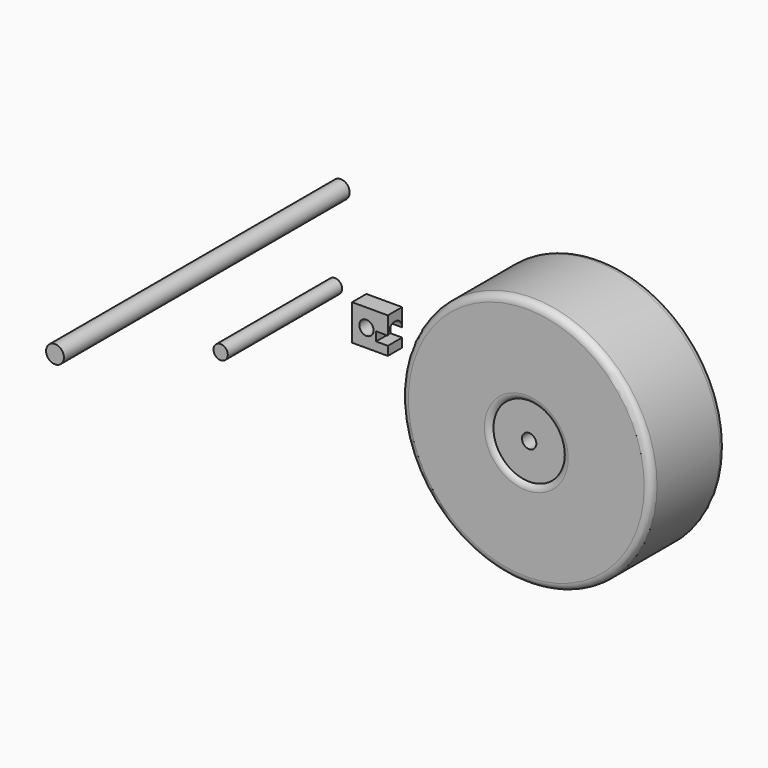
from build123d import *

# Parameters (mm, degrees)
F0_R     = 10
F0_R_2   = 2
F1_DEPTH = 12
F0_R_3   = 35
F2_DEPTH = 13
F4_R     = 2.5
F5_DEPTH = 100
F4_R_2   = 2
F6_DEPTH = 40
F4_W     = 3.3058956834
F4_H     = 1
F4_H_2   = 2.5
F7_DEPTH = 2.5


# Not quite as in the source:
# - a fillet or chamfer that OpenCascade refuses, or shapes differently, is made with other operations: its cross-section is extruded or revolved along the edge and cut away or added


with BuildPart() as f1:
    # F0 (on Front) → F1 (new body, symmetric)
    with BuildSketch(Plane.XZ):
        Circle(F0_R)
        Circle(F0_R_2, mode=Mode.SUBTRACT)
    extrude(amount=F1_DEPTH, both=True)

    # F0 (on Front) → F2 (join, symmetric)
    with BuildSketch(Plane.XZ):
        Circle(F0_R_3)
        Circle(F0_R, mode=Mode.SUBTRACT)
    extrude(amount=F2_DEPTH, both=True)

    # F3: fillet of radius 2 on 4 edges, made by hand

    # F3_s1 → F3_t2 (revolve, cut)
    with BuildSketch(Plane.XY):
        with BuildLine():
            ThreePointArc((11.7320508076, 13), (10.7320508076, 12.7320508076), (10, 12))
            Line((10, 12), (10, 13))
            Line((10, 13), (11.7320508076, 13))
        make_face()
    revolve(axis=Axis((0, 13, 0), (0, -1, 0)), mode=Mode.SUBTRACT)

    # F3_s3 → F3_t4 (revolve, cut)
    with BuildSketch(Plane.XY):
        with BuildLine():
            ThreePointArc((11.7320508076, -13), (10.7320508076, -12.7320508076), (10, -12))
            Line((10, -12), (10, -13))
            Line((10, -13), (11.7320508076, -13))
        make_face()
    revolve(axis=Axis((0, -13, 0), (0, -1, 0)), mode=Mode.SUBTRACT)

    # F3_s5 → F3_t6 (revolve, cut)
    with BuildSketch(Plane.XY):
        with BuildLine():
            ThreePointArc((35, -11), (34.4142135624, -12.4142135624), (33, -13))
            Line((33, -13), (35, -13))
            Line((35, -13), (35, -11))
        make_face()
    revolve(axis=Axis((0, -13, 0), (0, -1, 0)), mode=Mode.SUBTRACT)

    # F3_s7 → F3_t8 (revolve, cut)
    with BuildSketch(Plane.XY):
        with BuildLine():
            ThreePointArc((35, 11), (34.4142135624, 12.4142135624), (33, 13))
            Line((33, 13), (35, 13))
            Line((35, 13), (35, 11))
        make_face()
    revolve(axis=Axis((0, 13, 0), (0, -1, 0)), mode=Mode.SUBTRACT)


with BuildPart() as f5:
    # F4 (on Front) → F5 (new body)
    with BuildSketch(Plane.XZ):
        with Locations((-62.3413799527, 36.9166958029)):
            Circle(F4_R)
    extrude(amount=F5_DEPTH)


with BuildPart() as f6:
    # F4 (on Front) → F6 (new body)
    with BuildSketch(Plane.XZ):
        with Locations((-63.968997372, 12.5027095192)):
            Circle(F4_R_2)
    extrude(amount=F6_DEPTH)


with BuildPart() as f7:
    # F4 (on Front) → F7 (new body, symmetric)
    with BuildSketch(Plane.XZ):
        Polygon((-47.1659764079, 10.2858506218), (-47.1659764079, 11.7858506218), (-57.1659764079, 11.7858506218), (-57.1659764079, 10.2858506218), (-50.4718720913, 10.2858506218), align=None)
        Polygon((-50.4718720913, 10.2858506218), (-57.1659764079, 10.2858506218), (-57.1659764079, 3.2858506218), (-50.4718720913, 3.2858506218), (-50.4718720913, 4.2858506218), (-50.4718720913, 6.7858506218), (-50.4718720913, 9.2858506218), align=None)
        with Locations((-53.1659764079, 6.7858506218)):
            Circle(F4_R_2, mode=Mode.SUBTRACT)
        Polygon((-50.4718720913, 3.2858506218), (-57.1659764079, 3.2858506218), (-57.1659764079, 1.7858506218), (-47.1659764079, 1.7858506218), (-47.1659764079, 3.2858506218), align=None)
        with Locations((-48.8189242496, 9.7858506218)):
            Rectangle(F4_W, F4_H)
        with Locations((-48.8189242496, 8.0358506218)):
            Rectangle(F4_W, F4_H_2)
        with Locations((-48.8189242496, 3.7858506218)):
            Rectangle(F4_W, F4_H)
    extrude(amount=F7_DEPTH, both=True)

    # F4 (on Front) → F8 (revolve, cut)
    with BuildSketch(Plane.XZ):
        with Locations((-48.8189242496, 5.5358506218)):
            Rectangle(F4_W, F4_H_2)
    revolve(axis=Axis((-48.8189242496, 0, 6.7858506218), (1, 0, 0)), mode=Mode.SUBTRACT)


solid = Compound([f1.part, f5.part, f6.part, f7.part])
